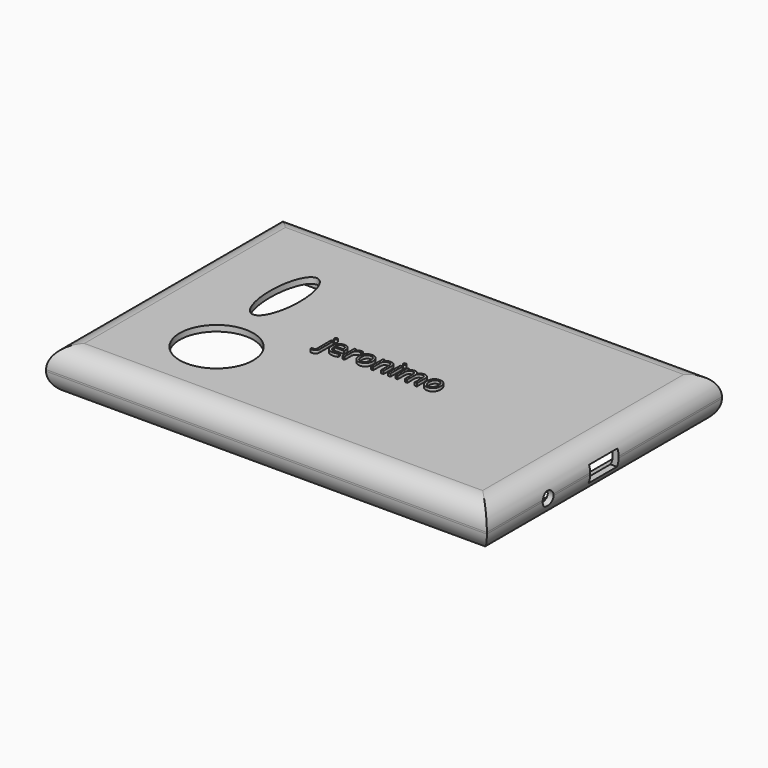
from build123d import *

# Parameters (mm, degrees)
F0_W         = 150
F0_H         = 100
F1_DEPTH     = 15
F2_R         = 7.2426406871
F3_T         = -2
F4_R         = 12.5303653763
F5_DEPTH     = 25
F6_W         = 12.0983086526
F6_H         = 5.5899326167
F6_R         = 2.3345525608
F7_DEPTH     = 25
F8_TEXT_SIZE = 9.598572635
F9_DEPTH     = 1


# Not quite as in the source:
# - a shell that OpenCascade refuses in one call is made with other operations: the cavity is built on its own and cut out
# - Text() gives the source's letters only with a copy of the font that has no kerning and outlines rounded to 1/6400 em; it was checked with that copy


with BuildPart() as f1:
    # F0 (on Top) → F1 (new body)
    with BuildSketch(Plane.XY):
        Rectangle(F0_W, F0_H)
    extrude(amount=F1_DEPTH)

    # F2
    f2_edges = [f1.edges().sort_by_distance(p)[0] for p in [
        (0, -50, 15),
        (75, 0, 15),
        (0, 50, 15),
        (-75, 0, 15),
        (0, -50, 0),
        (0, 50, 0),
        (-75, 0, 0),
        (75, 0, 0),
    ]]
    fillet(f2_edges, radius=F2_R)

    # F3: a shell. OpenCascade refuses it in one call, so the cavity is built on its own and cut out:
    # the body offset inwards by the wall thickness, plus a prism from it out through each open face.
    f3_core = offset(f1.part, amount=F3_T, mode=Mode.PRIVATE)
    f3_exits = [f3_core.faces().sort_by_distance(p)[0] for p in [
        (0, 0, 2),
    ]]
    add(f3_core, mode=Mode.SUBTRACT)
    extrude(f3_exits, amount=-F3_T, mode=Mode.SUBTRACT)

    # F4 (on face) → F5 (cut)
    with BuildSketch(Plane.XY.offset(15)):
        with Locations((-39.1542494301, -22.2912859898)):
            Circle(F4_R)
        with BuildLine():
            add(Edge.make_bspline(
                [(-43.1071929634, 25.2120271325), (-51.833092548, 25.2120271325), (-47.4701427557, 4.9816849642), (-43.1071929634, -15.2486572042), (-38.744243171, 4.9816849642), (-34.3812933787, 25.2120271325), (-43.1071929634, 25.2120271325)],
                knots=[0, 0, 0, 2.0943951024, 2.0943951024, 4.1887902048, 4.1887902048, 6.2831853072, 6.2831853072, 6.2831853072], degree=2, weights=[1, 0.5, 1, 0.5, 1, 0.5, 1]))
        make_face()
    extrude(amount=-F5_DEPTH, mode=Mode.SUBTRACT)

    # F6 (on face) → F7 (cut)
    with BuildSketch(Plane.YZ.offset(75)):
        with Locations((0, 7.2426406871)):
            Rectangle(F6_W, F6_H)
        with Locations((-23.9191334695, 7.2426406871)):
            Circle(F6_R)
    extrude(amount=-F7_DEPTH, mode=Mode.SUBTRACT)

    # F8 (on face) → F9 (join)
    with BuildSketch(Plane.XY.offset(15)):
        with Locations((-17.2867402434, -6.9109722972)):
            Text('jeronimo', F8_TEXT_SIZE, font='Open Sans', text_align=(TextAlign.LEFT, TextAlign.BOTTOM))
    extrude(amount=F9_DEPTH)


solid = f1.part
